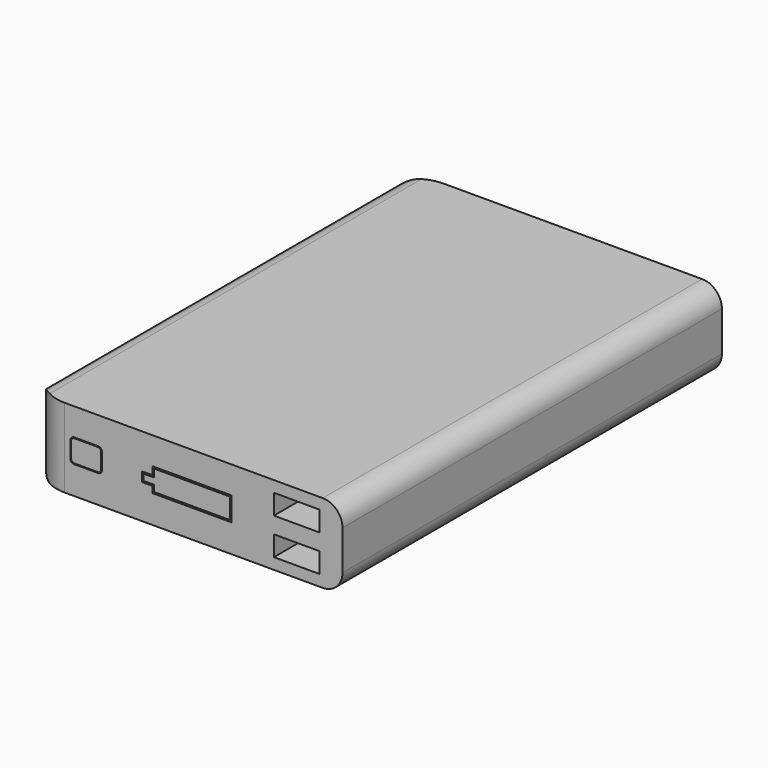
from build123d import *

# Parameters (mm, degrees)
F1_DEPTH    = 152.4
F2_T1_DEPTH = 74.0210244843
F3_T1_DEPTH = 74.041
F4_W        = 14.6846622229
F4_H        = 6.4612496644
F5_DEPTH    = 12.7
F7_DEPTH    = 2.54
F9_DEPTH    = 2.54


# Not quite as in the source:
# - a fillet or chamfer that OpenCascade refuses, or shapes differently, is made with other operations: its cross-section is extruded or revolved along the edge and cut away or added


with BuildPart() as f1:
    # F0 (on Front) → F1 (new body)
    with BuildSketch(Plane.XZ):
        with BuildLine():
            Line((0, 19.05), (0, 6.35))
            ThreePointArc((0, 6.35), (1.8598719395, 1.8598719395), (6.35, 0))
            Line((6.35, 0), (95.25, 0))
            ThreePointArc((95.25, 0), (99.7401280605, 1.8598719395), (101.6, 6.35))
            Line((101.6, 6.35), (101.6, 19.05))
            ThreePointArc((101.6, 19.05), (99.7401280605, 23.5401280605), (95.25, 25.4))
            Line((95.25, 25.4), (6.35, 25.4))
            ThreePointArc((6.35, 25.4), (1.8598719395, 23.5401280605), (0, 19.05))
        make_face()
    extrude(amount=F1_DEPTH)

    # F2: fillet of radius 12.2642048969 on 1 edges, made by hand

    # F2_s2 → F2_t1 (cut)
    with BuildSketch(Plane.XY.offset(-24.3105122421)):
        with BuildLine():
            ThreePointArc((0, -140.1357951031), (3.5921024484, -148.8078975516), (12.2642048969, -152.4))
            Line((12.2642048969, -152.4), (0, -152.4))
            Line((0, -152.4), (0, -140.1357951031))
        make_face()
    extrude(amount=F2_T1_DEPTH, mode=Mode.SUBTRACT)

    # F3: fillet of radius 12.2682 on 1 edges, made by hand

    # F3_s2 → F3_t1 (cut)
    with BuildSketch(Plane.XY.offset(-24.3205)):
        with BuildLine():
            ThreePointArc((12.2682, 0), (3.593272587, -3.593272587), (0, -12.2682))
            Line((0, -12.2682), (0, 0))
            Line((0, 0), (12.2682, 0))
        make_face()
    extrude(amount=F3_T1_DEPTH, mode=Mode.SUBTRACT)

    # F4 (on face) → F5 (cut)
    with BuildSketch(Plane.XZ.offset(152.4)):
        with Locations((86.9044545794, 18.573864289)):
            Rectangle(F4_W, F4_H)
        with Locations((86.904451251, 6.8261355627)):
            Rectangle(F4_W, F4_H)
    extrude(amount=-F5_DEPTH, mode=Mode.SUBTRACT)

    # F6 (on face) → F7 (cut)
    with BuildSketch(Plane.XZ.offset(152.4)):
        Polygon((40.5169758041, 14.0975351255), (37.2149758041, 14.0975351255), (37.2149758041, 11.0495351255), (40.5169758041, 11.0495351255), (40.5169758041, 9.0060108787), (65.9169758041, 9.0060108787), (65.9169758041, 16.6260108787), (40.5169758041, 16.6260108787), align=None)
        Polygon((65.4089756118, 16.1180106864), (65.4089756118, 9.514011071), (41.0249759964, 9.514011071), (41.0249759964, 11.5575353178), (37.7229759964, 11.5575353178), (37.7229759964, 13.5895349332), (41.0249759964, 13.5895349332), (41.0249759964, 16.1180106864), align=None, mode=Mode.SUBTRACT)
    extrude(amount=-F7_DEPTH, mode=Mode.SUBTRACT)

    # F8 (on face) → F9 (cut)
    with BuildSketch(Plane.XZ.offset(152.4)):
        with BuildLine():
            Line((23.0576487401, 16.6260112998), (15.4376487401, 16.6260112998))
            ThreePointArc((15.4376487401, 16.6260112998), (14.539623128, 16.2540369119), (14.1676487401, 15.3560112998))
            Line((14.1676487401, 15.3560112998), (14.1676487401, 10.2760112998))
            ThreePointArc((14.1676487401, 10.2760112998), (14.539623128, 9.3779856877), (15.4376487401, 9.0060112998))
            Line((15.4376487401, 9.0060112998), (23.0576487401, 9.0060112998))
            ThreePointArc((23.0576487401, 9.0060112998), (23.9556743522, 9.3779856877), (24.3276487401, 10.2760112998))
            Line((24.3276487401, 10.2760112998), (24.3276487401, 15.3560112998))
            ThreePointArc((24.3276487401, 15.3560112998), (23.9556743522, 16.2540369119), (23.0576487401, 16.6260112998))
        make_face()
        with BuildLine():
            ThreePointArc((14.4295694742, 15.3560112998), (14.7248290552, 16.0688309847), (15.4376487401, 16.3640905657))
            Line((15.4376487401, 16.3640905657), (23.0576487401, 16.3640905657))
            ThreePointArc((23.0576487401, 16.3640905657), (23.770468425, 16.0688309847), (24.0657280061, 15.3560112998))
            Line((24.0657280061, 15.3560112998), (24.0657280061, 10.2760112998))
            ThreePointArc((24.0657280061, 10.2760112998), (23.770468425, 9.5631916149), (23.0576487401, 9.2679320338))
            Line((23.0576487401, 9.2679320338), (15.4376487401, 9.2679320338))
            ThreePointArc((15.4376487401, 9.2679320338), (14.7248290552, 9.5631916149), (14.4295694742, 10.2760112998))
            Line((14.4295694742, 10.2760112998), (14.4295694742, 15.3560112998))
        make_face(mode=Mode.SUBTRACT)
    extrude(amount=-F9_DEPTH, mode=Mode.SUBTRACT)


solid = f1.part
